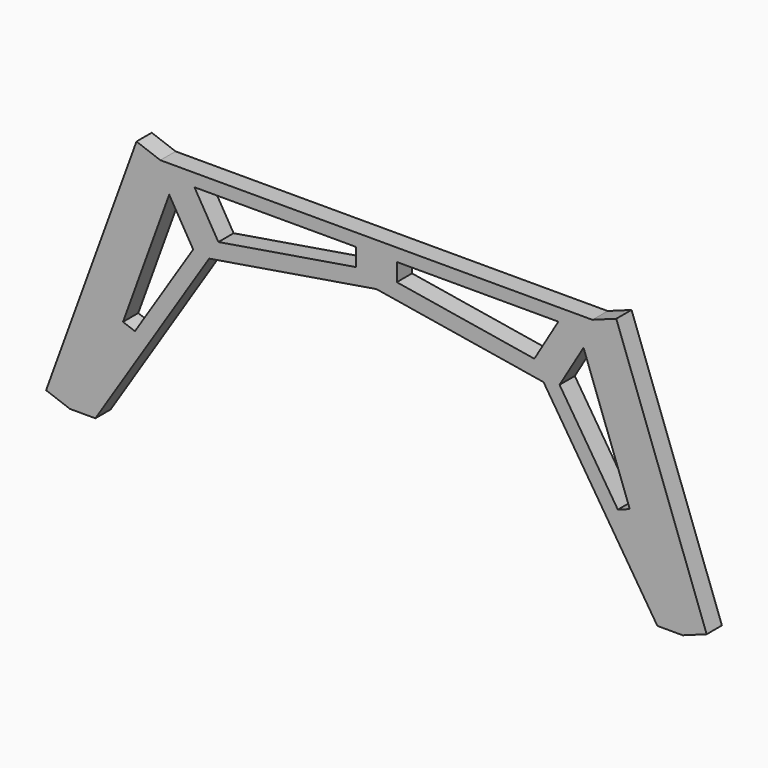
from build123d import *

# Parameters (mm, degrees)
F2_DEPTH = 19.05


# Not quite as in the source:
# - a variable given as a bare number and used for a length is read in inches; the dataset says mm whatever the document's units were


with BuildPart() as f2:
    # F1 (on Front) → F2 (new body)
    with BuildSketch(Plane.XZ):
        Polygon((215.9, 0), (0, 0), (-215.9, 0), (-306.2480410609, -248.2292027068), (-280.8480410609, -248.2292027068), (-167.1250061285, -70.7126014387), (0, -43.18), (167.1250061285, -70.7126014387), (280.8480410609, -248.2292027068), (306.2480410609, -248.2292027068), align=None)
        Polygon((-253.2563468183, -154.4156124752), (-207.0382383225, -27.4324030132), (-183.0905760207, -67.8622134293), (-241.3222505343, -158.7592682954), align=None, mode=Mode.SUBTRACT)
        Polygon((-181.84793878, -12.7), (-20.4141870137, -12.7), (-20.4141870137, -30.48), (-157.9002764782, -53.1298104161), align=None, mode=Mode.SUBTRACT)
        Polygon((183.0905760207, -67.8622134293), (207.0382383225, -27.4324030132), (253.2563468183, -154.4156124752), (241.3222505343, -158.7592682954), align=None, mode=Mode.SUBTRACT)
        Polygon((157.9002764782, -53.1298104161), (20.4141870137, -30.48), (20.4141870137, -12.7), (181.84793878, -12.7), align=None, mode=Mode.SUBTRACT)
        Polygon((-306.2480410609, -248.2292027068), (-215.9, 0), (-239.768192568, 8.6873116405), (-330.1162336289, -239.5418910663), align=None)
        Polygon((239.768192568, 8.6873116405), (215.9, 0), (306.2480410609, -248.2292027068), (330.1162336289, -239.5418910663), align=None)
    extrude(amount=F2_DEPTH)


solid = f2.part
